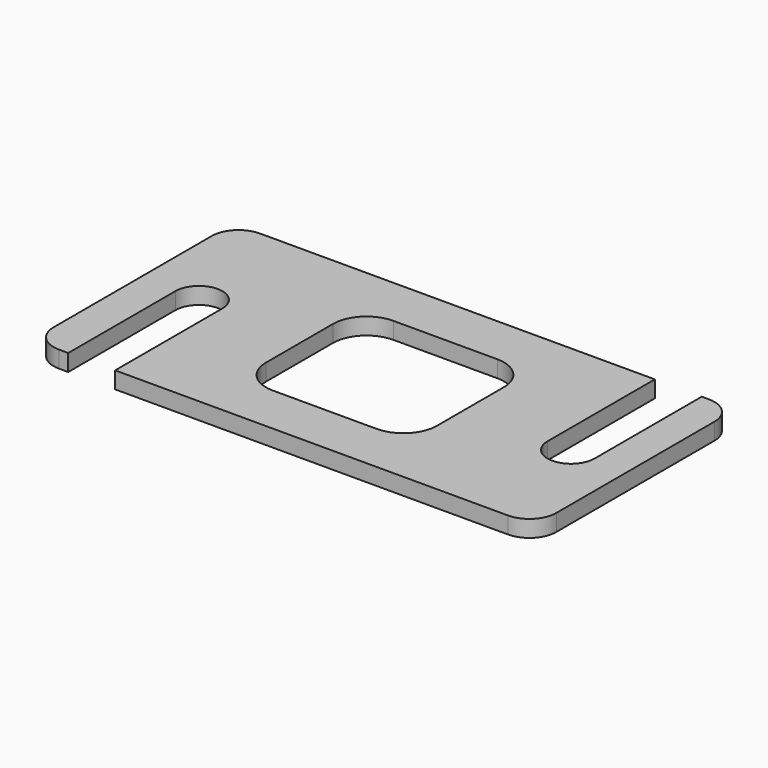
from build123d import *

# Parameters (mm, degrees)
F0_W     = 150
F0_H     = 75
F1_DEPTH = 5
F3_DEPTH = 282
F4_DEPTH = 5.001
F5_W     = 51.0268339871
F5_H     = 45
F6_DEPTH = 5.001
F7_R     = 10
F8_R     = 8


# Not quite as in the source:
# - an extrude ends at something that could not be found from the text; its depth is read off the source's solid


with BuildPart() as f1:
    # F0 (on Top) → F1 (new body)
    with BuildSketch(Plane.XY):
        with Locations((-33.9150866494, -108.2351529738)):
            Rectangle(F0_W, F0_H)
    extrude(amount=F1_DEPTH)

    # F2 (on Top) → F3 (cut, through all)
    with BuildSketch(Plane.XY):
        with BuildLine():
            Line((-98.1348048404, -105.7351529738), (-98.1348048404, -145.7351529738))
            Line((-98.1348048404, -145.7351529738), (-84.1348048404, -145.7351529738))
            Line((-84.1348048404, -145.7351529738), (-84.1348048404, -105.7351529738))
            ThreePointArc((-84.1348048404, -105.7351529738), (-91.1348048404, -98.7351529738), (-98.1348048404, -105.7351529738))
        make_face()
        with BuildLine():
            Line((30.8920291467, -110.7351529738), (30.8920291467, -70.7351529738))
            Line((30.8920291467, -70.7351529738), (16.8920291467, -70.7351529738))
            Line((16.8920291467, -70.7351529738), (16.8920291467, -110.7351529738))
            ThreePointArc((16.8920291467, -110.7351529738), (23.8920291467, -117.7351529738), (30.8920291467, -110.7351529738))
        make_face()
    extrude(amount=-F3_DEPTH, mode=Mode.SUBTRACT)

    # F2 (on Top) → F4 (cut, through all)
    with BuildSketch(Plane.XY):
        with BuildLine():
            Line((-98.1348048404, -105.7351529738), (-98.1348048404, -145.7351529738))
            Line((-98.1348048404, -145.7351529738), (-84.1348048404, -145.7351529738))
            Line((-84.1348048404, -145.7351529738), (-84.1348048404, -105.7351529738))
            ThreePointArc((-84.1348048404, -105.7351529738), (-91.1348048404, -98.7351529738), (-98.1348048404, -105.7351529738))
        make_face()
        with BuildLine():
            Line((30.8920291467, -110.7351529738), (30.8920291467, -70.7351529738))
            Line((30.8920291467, -70.7351529738), (16.8920291467, -70.7351529738))
            Line((16.8920291467, -70.7351529738), (16.8920291467, -110.7351529738))
            ThreePointArc((16.8920291467, -110.7351529738), (23.8920291467, -117.7351529738), (30.8920291467, -110.7351529738))
        make_face()
    extrude(amount=F4_DEPTH, mode=Mode.SUBTRACT)

    # F5 (on face) → F6 (cut, through all)
    with BuildSketch(Plane.XY.offset(5)):
        with Locations((-33.6213878469, -108.2351529738)):
            Rectangle(F5_W, F5_H)
    extrude(amount=-F6_DEPTH, mode=Mode.SUBTRACT)

    # F7
    f7_edges = [f1.edges().sort_by_distance(p)[0] for p in [
        (-8.107971, -85.735153, 2.5),
        (-8.107971, -130.735153, 2.5),
        (-59.134805, -130.735153, 2.5),
        (-59.134805, -85.735153, 2.5),
    ]]
    fillet(f7_edges, radius=F7_R)

    # F8
    f8_edges = [f1.edges().sort_by_distance(p)[0] for p in [
        (41.084913, -145.735153, 2.5),
        (41.084913, -70.735153, 2.5),
        (-108.915087, -70.735153, 2.5),
        (-108.915087, -145.735153, 2.5),
    ]]
    fillet(f8_edges, radius=F8_R)


solid = f1.part
